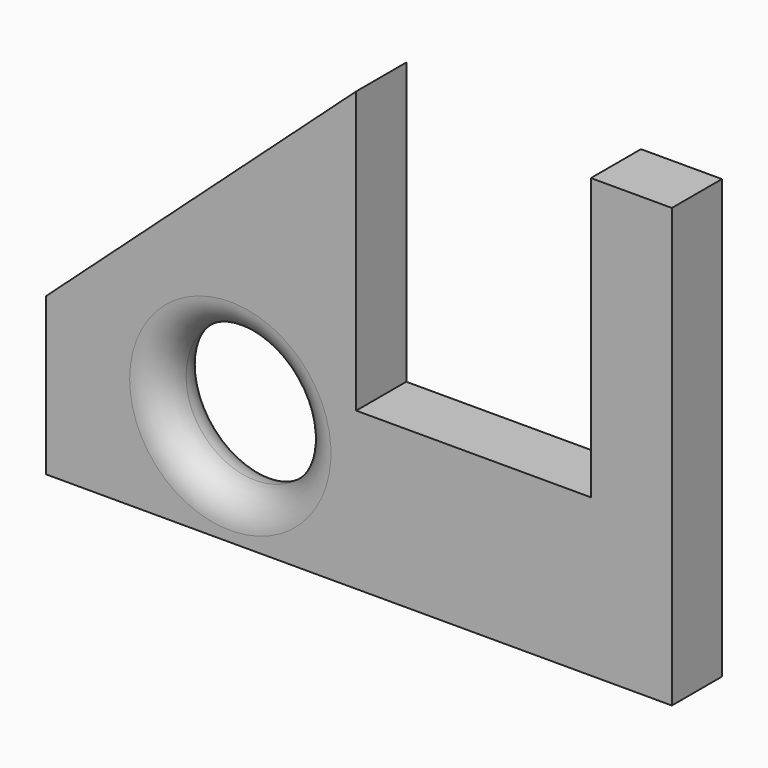
from build123d import *

# Parameters (mm, degrees)
F1_DEPTH = 25.4
F2_R     = 28.1548982212
F3_DEPTH = 25.401
F4_R     = 12.69999


# Not quite as in the source:
# - a fillet or chamfer is up to 0.001 mm smaller than in the source, because OpenCascade refuses the exact size


with BuildPart() as f1:
    # F0 (on Front) → F1 (new body)
    with BuildSketch(Plane.XZ):
        Polygon((0, 63.7160863788), (0, 0), (254, 0), (254, 177.8), (221.1352040053, 177.8), (221.1352040053, 63.7160863788), (125.8798138147, 63.7160863788), (125.8798138147, 177.8), align=None)
    extrude(amount=F1_DEPTH)

    # F2 (on face) → F3 (cut, through all)
    with BuildSketch(Plane(origin=(0, 0, 0), x_dir=(-1, 0, 0), z_dir=(0, 1, 0))):
        with Locations((-74.7735798359, 45.1450571418)):
            Circle(F2_R)
    extrude(amount=-F3_DEPTH, mode=Mode.SUBTRACT)

    # F4 (radius 12.7 in the source; OpenCascade refuses exactly that, so slightly less here)
    f4_edges = [f1.edges().sort_by_distance(p)[0] for p in [
        (102.928478, 0, 45.145057),
        (102.928478, -25.4, 45.145057),
    ]]
    fillet(f4_edges, radius=F4_R)


solid = f1.part
